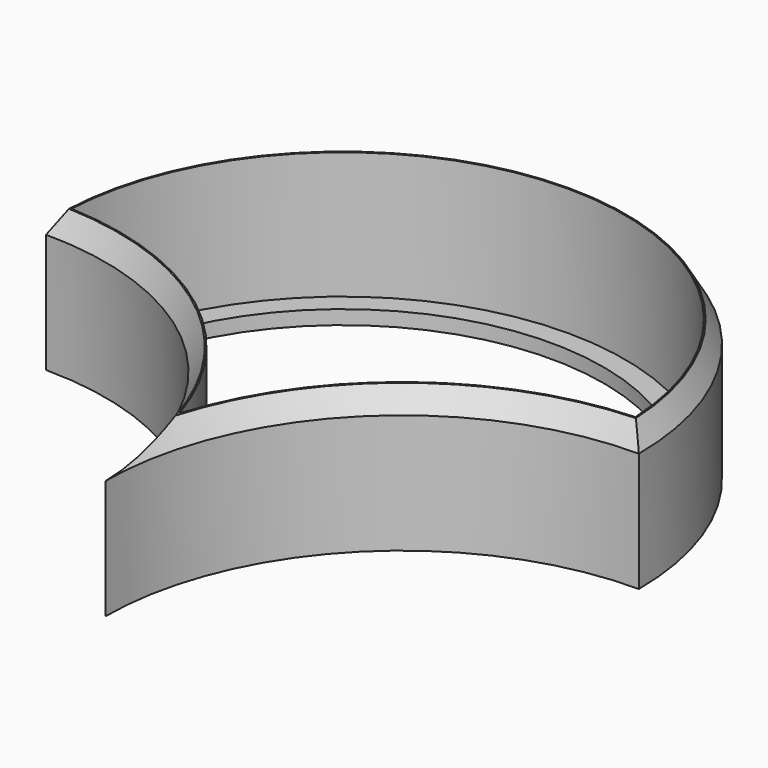
from build123d import *

# Parameters (mm, degrees)
F1_DEPTH    = 25.4
F2_T        = -2.54
F3_T2_ANGLE = 202.0417037701
F3_T4_ANGLE = 119.7204573229
F3_T6_ANGLE = 119.7204573229
F5_DEPTH    = 2.54


# Not quite as in the source:
# - a fillet or chamfer that OpenCascade refuses, or shapes differently, is made with other operations: its cross-section is extruded or revolved along the edge and cut away or added


with BuildPart() as f1:
    # F0 (on Top) → F1 (new body)
    with BuildSketch(Plane.XY):
        with BuildLine():
            ThreePointArc((-53.34, 0), (-15.6229242915, -15.6229242915), (0, -53.34))
            ThreePointArc((0, -53.34), (15.6229242915, -15.6229242915), (53.34, 0))
            ThreePointArc((53.34, 0), (0, 53.34), (-53.34, 0))
        make_face()
    extrude(amount=F1_DEPTH)

    # F2
    f2_openings = [f1.faces().sort_by_distance(p)[0] for p in [
        (0, 15.223138, 25.4),
    ]]
    offset(amount=F2_T, openings=f2_openings)

    # F3: chamfer of 2.286 x 3.9594681461 on 3 edges, made by hand

    # F3_s1 → F3_t2 (revolve, cut)
    with BuildSketch(Plane(origin=(0, 0, 0), x_dir=(0, 0, 1), z_dir=(-0.1911662303, -0.9815576766, 0))):
        Polygon((21.4405318539, -53.34), (25.4, -51.054), (25.4, -53.34), align=None)
    revolve(axis=Axis((0, 0, 25.4), (0, 0, 1)), revolution_arc=F3_T2_ANGLE, mode=Mode.SUBTRACT)

    # F3_s3 → F3_t4 (revolve, cut)
    with BuildSketch(Plane(origin=(-61.3926477335, -11.9419473665, 0), x_dir=(0, 0, 1), z_dir=(-0.9816019423, -0.190938804, 0))):
        Polygon((21.4405318539, 11.1660282003), (25.4, 13.4520282003), (25.4, 11.1660282003), align=None)
    revolve(axis=Axis((-53.34, -53.34, 25.4), (0, 0, -1)), revolution_arc=F3_T4_ANGLE, mode=Mode.SUBTRACT)

    # F3_s5 → F3_t6 (revolve, cut)
    with BuildSketch(Plane(origin=(21.6984854346, -64.0579906243, 0), x_dir=(0, 0, 1), z_dir=(0.3208259227, -0.9471381775, 0))):
        Polygon((21.4405318539, 19.9325043289), (25.4, 22.2185043289), (25.4, 19.9325043289), align=None)
    revolve(axis=Axis((53.34, -53.34, 25.4), (0, 0, -1)), revolution_arc=F3_T6_ANGLE, mode=Mode.SUBTRACT)

    # F4 (on face) → F5 (cut, through all)
    with BuildSketch(Plane(origin=(0, 0, 0), x_dir=(1, 0, 0), z_dir=(0, 0, -1))):
        with BuildLine():
            ThreePointArc((-46.6093067615, -5.9693067615), (0, -46.99), (46.6093067615, -5.9693067615))
            ThreePointArc((46.6093067615, -5.9693067615), (19.1861227863, 4.3868716907), (0, 26.5493206506))
            ThreePointArc((0, 26.5493206506), (-19.1861227863, 4.3868716907), (-46.6093067615, -5.9693067615))
        make_face()
    extrude(amount=-F5_DEPTH, mode=Mode.SUBTRACT)


solid = f1.part
